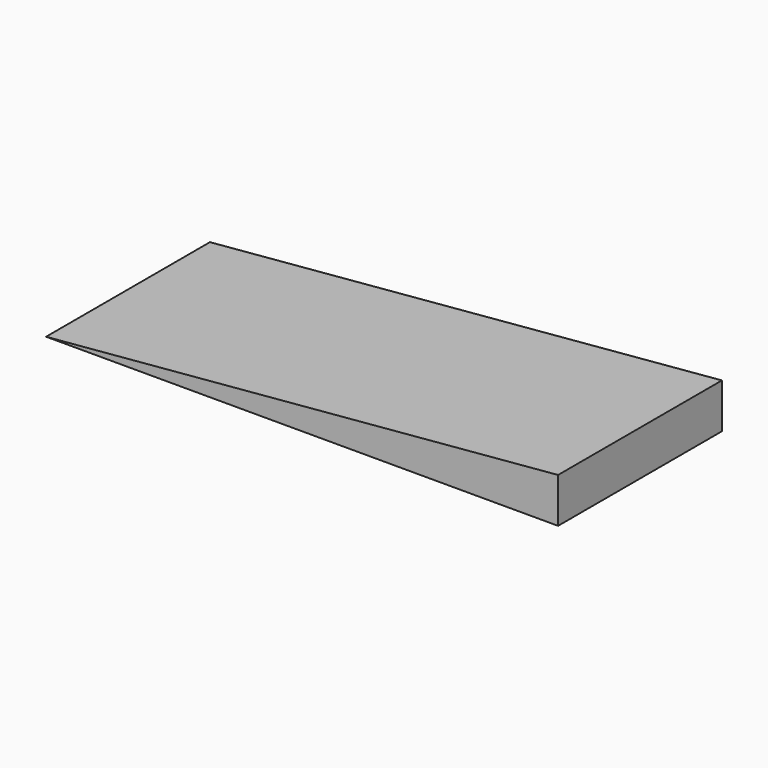
from build123d import *

# Parameters (mm, degrees)
F0_W        = 50
F0_H        = 20
F1_DEPTH    = 5
F2_T1_DEPTH = 317.1395350057


# Not quite as in the source:
# - a fillet or chamfer that OpenCascade refuses, or shapes differently, is made with other operations: its cross-section is extruded or revolved along the edge and cut away or added


with BuildPart() as f1:
    # F0 (on Top) → F1 (new body)
    with BuildSketch(Plane.XY):
        Rectangle(F0_W, F0_H)
    extrude(amount=F1_DEPTH)

    # F2: chamfer of 5 x 57.1502615138 on 1 edges, made by hand

    # F2_s2 → F2_t1 (cut)
    with BuildSketch(Plane.XZ.offset(-158.5697675028)):
        Polygon((-25, 0), (32.1502615138, 5), (-25, 5), align=None)
    extrude(amount=F2_T1_DEPTH, mode=Mode.SUBTRACT)


solid = f1.part
